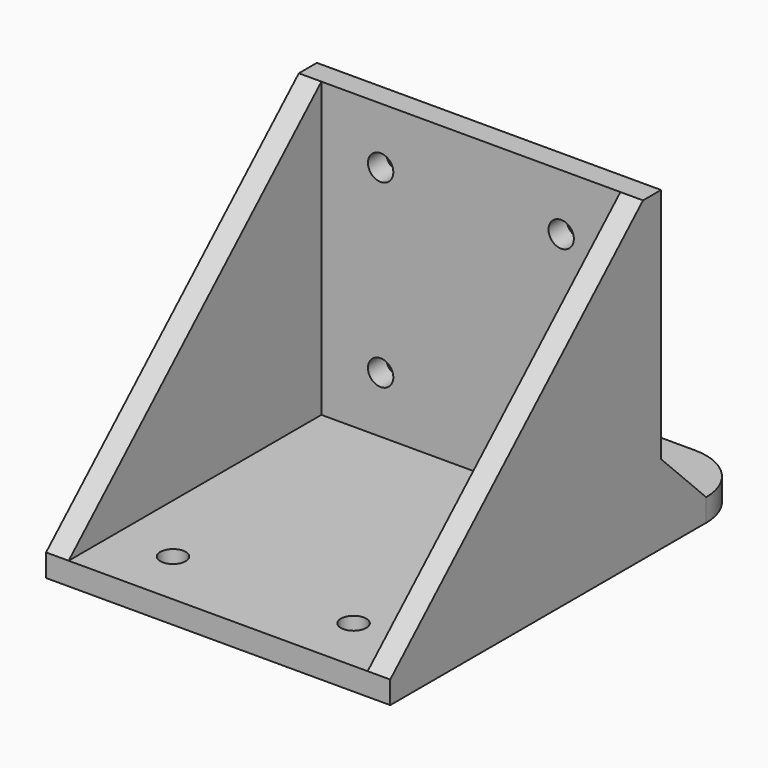
from build123d import *

# Parameters (mm, degrees)
F0_W      = 53
F0_H      = 60
F1_DEPTH  = 4
F2_W      = 53
F2_H      = 4
F3_DEPTH  = 52
F4_R      = 2.25
F5_DEPTH  = 56.001
F6_R      = 2.25
F7_DEPTH  = 60.001
F9_DEPTH  = 4
F11_DEPTH = 4
F12_W     = 61
F12_H     = 4
F13_DEPTH = 20
F14_R     = 2.25
F15_DEPTH = 4.001
F16_R     = 10


# Not quite as in the source:
# - a feature names something its author has since deleted; it is built from what else it names


with BuildPart() as f1:
    # F0 (on Top) → F1 (new body)
    with BuildSketch(Plane.XY):
        Rectangle(F0_W, F0_H)
    extrude(amount=F1_DEPTH)

    # F2 (on face) → F3 (join)
    with BuildSketch(Plane.XY.offset(4)):
        with Locations((0, 28)):
            Rectangle(F2_W, F2_H)
    extrude(amount=F3_DEPTH)

    # F4 (on face) → F5 (cut, through all)
    with BuildSketch(Plane(origin=(0, 0, 0), x_dir=(1, 0, 0), z_dir=(0, 0, -1))):
        with Locations((-16, 20)):
            Circle(F4_R)
        with Locations((16, 20)):
            Circle(F4_R)
    extrude(amount=-F5_DEPTH, mode=Mode.SUBTRACT)

    # F6 (on face) → F7 (cut, through all)
    with BuildSketch(Plane(origin=(0, 30, 0), x_dir=(-1, 0, 0), z_dir=(0, 1, 0))):
        with Locations((-16, 14)):
            Circle(F6_R)
        with Locations((-16, 46)):
            Circle(F6_R)
        with Locations((16, 14)):
            Circle(F6_R)
        with Locations((16, 46)):
            Circle(F6_R)
    extrude(amount=-F7_DEPTH, mode=Mode.SUBTRACT)

    # F8 (on face) → F9 (join)
    with BuildSketch(Plane.YZ.offset(26.5)):
        Polygon((30, 14), (30, 56), (26, 56), (-30, 4), (-30, 0), (30, 0), (30, 4), align=None)
        Polygon((40, 4), (30, 14), (30, 4), align=None)
    extrude(amount=F9_DEPTH)

    # F10 (on face) → F11 (join)
    with BuildSketch(Plane(origin=(-26.5, 0, 0), x_dir=(0, -1, 0), z_dir=(-1, 0, 0))):
        Polygon((-26, 56), (-30, 56), (-30, 14), (-30, 4), (-30, 0), (30, 0), (30, 4), align=None)
        Polygon((-30, 4), (-30, 14), (-40, 4), align=None)
    extrude(amount=F11_DEPTH)

    # F12 (on face) → F13 (join)
    with BuildSketch(Plane(origin=(0, 30, 0), x_dir=(-1, 0, 0), z_dir=(0, 1, 0))):
        with Locations((0, 2)):
            Rectangle(F12_W, F12_H)
    extrude(amount=F13_DEPTH)

    # F14 (on face) → F15 (cut, through all)
    with BuildSketch(Plane.XY.offset(4)):
        with Locations((16, 40)):
            Circle(F14_R)
        with Locations((-16, 40)):
            Circle(F14_R)
    extrude(amount=-F15_DEPTH, mode=Mode.SUBTRACT)

    # F16
    f16_edges = [f1.edges().sort_by_distance(p)[0] for p in [
        (30.5, 50, 2),
        (-30.5, 50, 2),
    ]]
    fillet(f16_edges, radius=F16_R)


solid = f1.part
